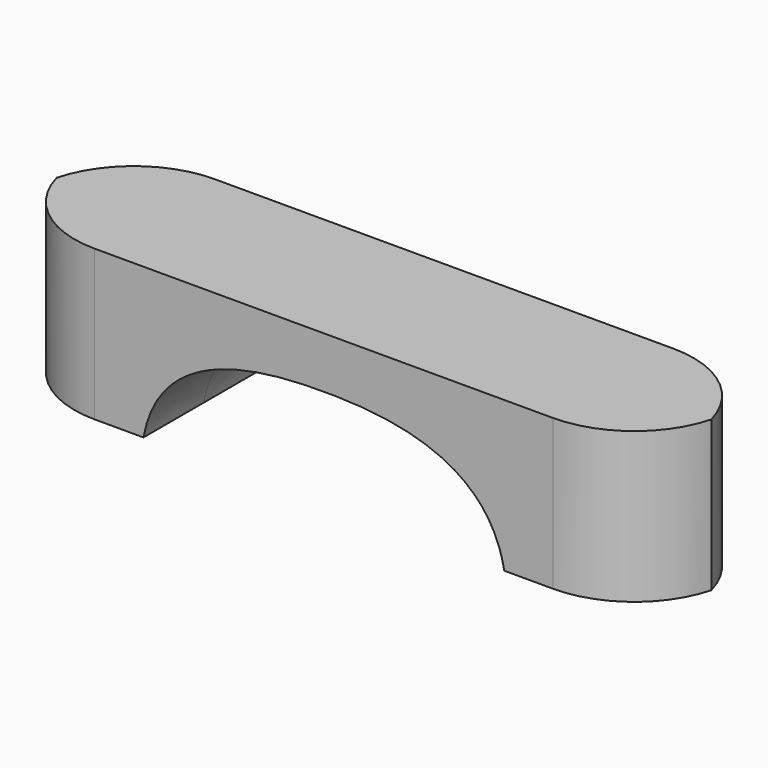
from build123d import *

# Parameters (mm, degrees)
F1_DEPTH    = 12.7
F2_T1_DEPTH = 111.249434278


# Not quite as in the source:
# - a fillet or chamfer that OpenCascade refuses, or shapes differently, is made with other operations: its cross-section is extruded or revolved along the edge and cut away or added


with BuildPart() as f1:
    # F0 (on Front) → F1 (new body, symmetric)
    with BuildSketch(Plane.XZ):
        with BuildLine():
            Line((-55.88, 0), (-30.48, 0))
            add(Edge.make_bspline(
                [(-30.48, 0), (-27.7506317943, 14.9127226323), (-11.670826003, 16.7281851172), (0, 16.7281851172)],
                knots=[0, 0, 0, 0, 34.7687011163, 34.7687011163, 34.7687011163, 34.7687011163], degree=3))
            add(Edge.make_bspline(
                [(30.48, 0), (27.7506317943, 14.9127226323), (11.670826003, 16.7281851172), (0, 16.7281851172)],
                knots=[0, 0, 0, 0, 34.7687011163, 34.7687011163, 34.7687011163, 34.7687011163], degree=3))
            Line((30.48, 0), (55.88, 0))
            Line((55.88, 0), (55.88, 25.4))
            Line((55.88, 25.4), (-55.88, 25.4))
            Line((-55.88, 25.4), (-55.88, 0))
        make_face()
    extrude(amount=F1_DEPTH, both=True)

    # F2: fillet of radius 17.1698868556 on 4 edges, made by hand

    # F2_s2 → F2_t1 (cut)
    with BuildSketch(Plane.XY.offset(-42.924717139)):
        with BuildLine():
            ThreePointArc((55.88, 4.4698868556), (50.8510565722, -7.6710565722), (38.7101131444, -12.7))
            Line((38.7101131444, -12.7), (55.88, -12.7))
            Line((55.88, -12.7), (55.88, 4.4698868556))
        make_face()
        with BuildLine():
            ThreePointArc((55.88, -4.4698868556), (50.8510565722, 7.6710565722), (38.7101131444, 12.7))
            Line((38.7101131444, 12.7), (55.88, 12.7))
            Line((55.88, 12.7), (55.88, -4.4698868556))
        make_face()
        with BuildLine():
            ThreePointArc((-55.88, 4.4698868556), (-50.8510565722, -7.6710565722), (-38.7101131444, -12.7))
            Line((-38.7101131444, -12.7), (-55.88, -12.7))
            Line((-55.88, -12.7), (-55.88, 4.4698868556))
        make_face()
        with BuildLine():
            ThreePointArc((-55.88, -4.4698868556), (-50.8510565722, 7.6710565722), (-38.7101131444, 12.7))
            Line((-38.7101131444, 12.7), (-55.88, 12.7))
            Line((-55.88, 12.7), (-55.88, -4.4698868556))
        make_face()
    extrude(amount=F2_T1_DEPTH, mode=Mode.SUBTRACT)


solid = f1.part
